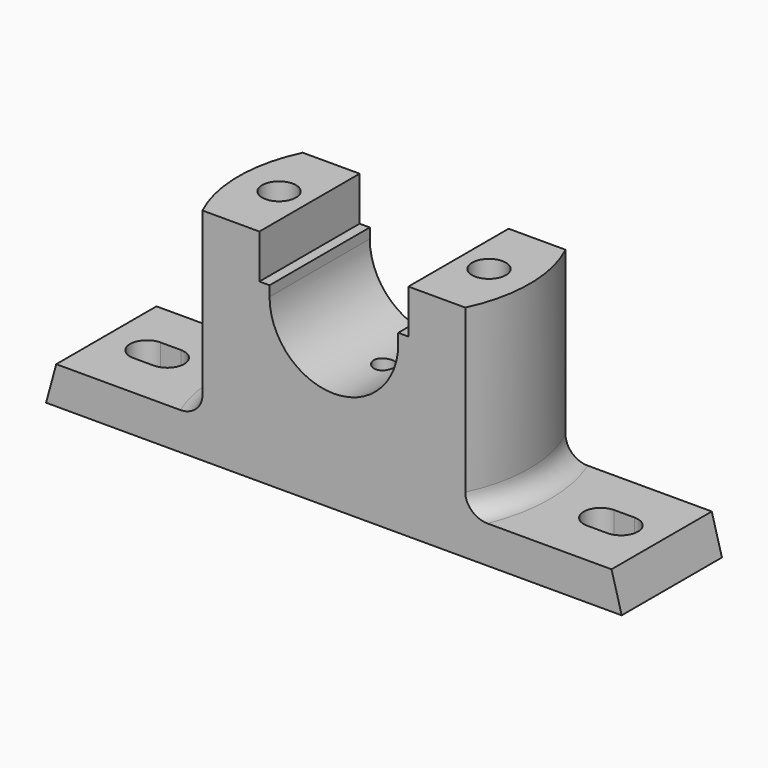
from build123d import *

# Parameters (mm, degrees)
F1_DEPTH  = 18.5
F3_DEPTH  = 54
F5_DEPTH  = 48.5
F6_R      = 5
F7_DEPTH  = 65.001
F8_W      = 12
F8_H      = 12
F9_DEPTH  = 8
F10_W     = 71
F10_H     = 2
F11_DEPTH = 11
F13_DEPTH = 11.001
F17_R     = 6


# Not quite as in the source:
# - a pattern or mirror of a feature is missing from the dataset's text; its kind, count and spacing are read off the source's solid


with BuildPart() as f1:
    # F0 (on Front) → F1 (new body, symmetric)
    with BuildSketch(Plane.XZ):
        Polygon((-82, 11), (-85, 0), (85, 0), (82, 11), align=None)
    extrude(amount=F1_DEPTH, both=True)

    # F2 (on face) → F3 (join)
    with BuildSketch(Plane.XY.offset(11)):
        with BuildLine():
            Line((38.8168777724, 18.5), (-38.8168777724, 18.5))
            ThreePointArc((-38.8168777724, 18.5), (-43, 0), (-38.8168777724, -18.5))
            Line((-38.8168777724, -18.5), (38.8168777724, -18.5))
            ThreePointArc((38.8168777724, -18.5), (43, 0), (38.8168777724, 18.5))
        make_face()
    extrude(amount=F3_DEPTH)

    # F4 (on Front) → F5 (cut, symmetric)
    with BuildSketch(Plane.XZ):
        with BuildLine():
            Line((22, 65), (-22, 65))
            Line((-22, 65), (-22, 52))
            Line((-22, 52), (-19, 52))
            Line((-19, 52), (-19, 49))
            ThreePointArc((-19, 49), (0, 30), (19, 49))
            Line((19, 49), (19, 52))
            Line((19, 52), (22, 52))
            Line((22, 52), (22, 65))
        make_face()
    extrude(amount=F5_DEPTH, both=True, mode=Mode.SUBTRACT)

    # F6 (on face) → F7 (cut, through all)
    with BuildSketch(Plane.XY.offset(65)):
        with Locations((-31, 0)):
            Circle(F6_R)
        with Locations((31, 0)):
            Circle(F6_R)
    extrude(amount=-F7_DEPTH, mode=Mode.SUBTRACT)

    # F8 (on face) → F9 (cut)
    with BuildSketch(Plane(origin=(0, 0, 0), x_dir=(1, 0, 0), z_dir=(0, 0, -1))):
        with Locations((-31, 0)):
            Rectangle(F8_W, F8_H)
        with Locations((31, 0)):
            Rectangle(F8_W, F8_H)
    extrude(amount=-F9_DEPTH, mode=Mode.SUBTRACT)

    # F10 (on Front) → F11 (cut, symmetric)
    with BuildSketch(Plane.XZ):
        with Locations((-39.5, 1)):
            Rectangle(F10_W, F10_H)
    f11 = extrude(amount=F11_DEPTH, both=True, mode=Mode.SUBTRACT)

    # F11_copies: F11 across plane
    add(f11.mirror(Plane(origin=(0, 0, 0), x_dir=(0, 0, 1), z_dir=(1, 0, 0))), mode=Mode.SUBTRACT)

    # F12 (on face) → F13 (cut, through all)
    with BuildSketch(Plane.XY.offset(11)):
        with BuildLine():
            ThreePointArc((-70, 5), (-75, 0), (-70, -5))
            Line((-70, -5), (-64, -5))
            ThreePointArc((-64, -5), (-59, 0), (-64, 5))
            Line((-64, 5), (-70, 5))
        make_face()
        with BuildLine():
            ThreePointArc((70, -5), (75, 0), (70, 5))
            Line((70, 5), (64, 5))
            ThreePointArc((64, 5), (59, 0), (64, -5))
            Line((64, -5), (70, -5))
        make_face()
    extrude(amount=-F13_DEPTH, mode=Mode.SUBTRACT)

    # F14 (on Front) → F15 (revolve, cut)
    with BuildSketch(Plane.XZ):
        Polygon((3, 31.8085759505), (0, 31.8085759505), (0, 22.1974181429), (3, 24), align=None)
    revolve(axis=Axis((0, 0, 27.0029970467), (0, 0, -1)), mode=Mode.SUBTRACT)

    # F14 (on Front) → F16 (revolve, cut)
    with BuildSketch(Plane.XZ):
        Polygon((3, 31.8085759505), (0, 31.8085759505), (0, 22.1974181429), (3, 24), align=None)
    revolve(axis=Axis((0, 0, 27.0029970467), (0, 0, -1)), mode=Mode.SUBTRACT)

    # F17
    f17_edges = [f1.edges().sort_by_distance(p)[0] for p in [
        (43, 0, 11),
        (-43, 0, 11),
    ]]
    fillet(f17_edges, radius=F17_R)


solid = f1.part
